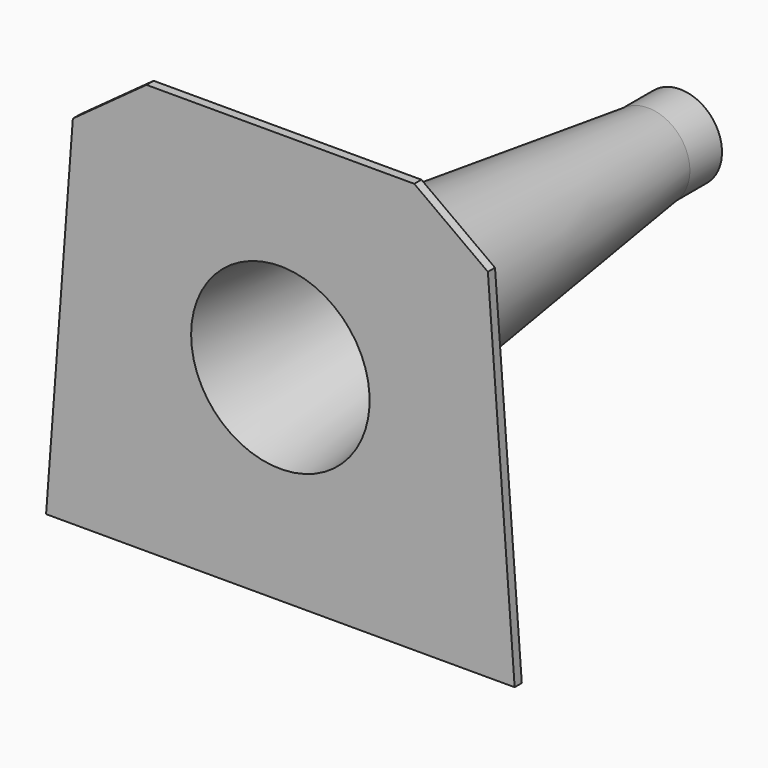
from build123d import *

# Parameters (mm, degrees)
F1_DEPTH = 2
F6_DEPTH = 3


with BuildPart() as f1:
    # F0 (on Front) → F1 (new body)
    with BuildSketch(Plane.XZ):
        Polygon((-52.5, -46), (52.5, -46), (46.5, 34), (30, 46), (-30, 46), (-46.5, 34), align=None)
    extrude(amount=-F1_DEPTH)

    # F2 (on Top) → F3 (revolve, cut)
    with BuildSketch(Plane.XY):
        Polygon((-20, 0), (0, 0), (0, 103), (-7.3619631902, 103), align=None)
    revolve(axis=Axis((0, 81.5, 0), (0, -1, 0)), mode=Mode.SUBTRACT)

    # F2 (on Top) → F4 (revolve)
    with BuildSketch(Plane.XY):
        Polygon((-22, 0), (-20, 0), (-7.3619631902, 103), (-9.3619631902, 103), align=None)
        Polygon((-9.3619631902, 103), (-7.3619631902, 103), (-7.3619631902, 112), (-8.2576687117, 112), align=None)
        Polygon((-9.3619631902, 112), (-9.3619631902, 103), (-8.2576687117, 112), align=None)
    revolve(axis=Axis((0, 2, 0), (0, -1, 0)))

    # F5 (on face) → F6 (join)
    with BuildSketch(Plane(origin=(0, 112, 0), x_dir=(-1, 0, 0), z_dir=(0, 1, 0))):
        with BuildLine():
            Line((-6.2, -3.9696979751), (-6.2, 0))
            Line((-6.2, 0), (-6.2, 3.9696979751))
            ThreePointArc((-6.2, 3.9696979751), (-7.3619631902, 0), (-6.2, -3.9696979751))
        make_face()
        with BuildLine():
            Line((6.0885886352, 4.1385493165), (6.2, 0))
            Line((6.2, 0), (6.3024315003, -3.8049782124))
            ThreePointArc((6.3024315003, -3.8049782124), (7.0921354587, -1.9748712995), (7.3619631902, 0))
            ThreePointArc((7.3619631902, 0), (7.0364219397, 2.1650100001), (6.0885886352, 4.1385493165))
        make_face()
    extrude(amount=-F6_DEPTH)


solid = f1.part
